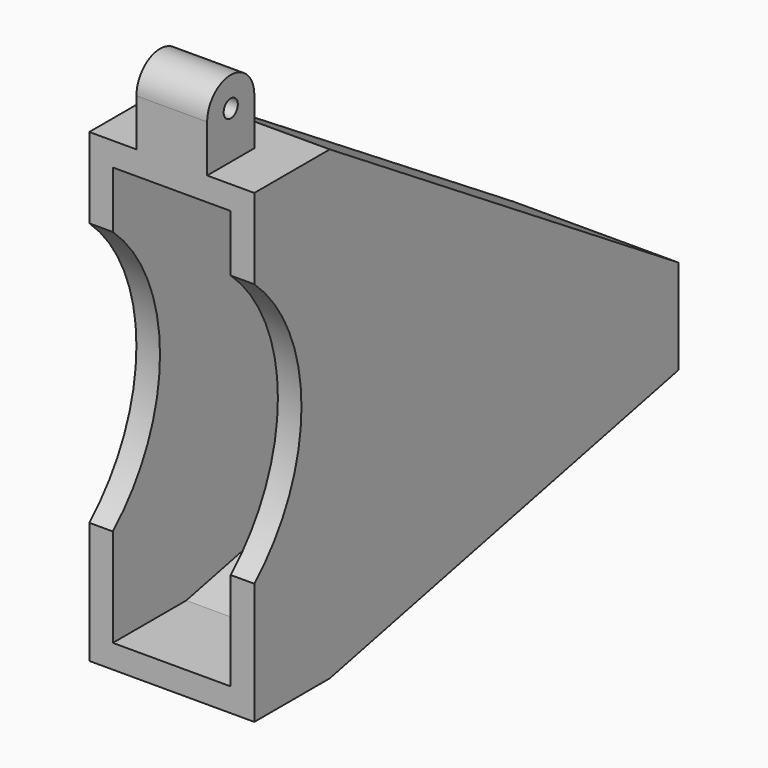
from build123d import *

# Parameters (mm, degrees)
F1_DEPTH = 7
F2_T     = -2
F3_R     = 0.75
F4_DEPTH = 3


# Not quite as in the source:
# - a feature names something its author has since deleted; it is built from what else it names


with BuildPart() as f1:
    # F0 (on Right) → F1 (new body, symmetric)
    with BuildSketch(Plane.YZ):
        with BuildLine():
            Line((45, 8), (45, 16))
            Line((45, 16), (8, 39.5))
            Line((8, 39.5), (0, 39.5))
            Line((0, 39.5), (0, 32.6803398875))
            ThreePointArc((0, 32.6803398875), (5, 21.5), (0, 10.3196601125))
            Line((0, 10.3196601125), (0, 0))
            Line((0, 0), (8, 0))
            Line((8, 0), (45, 8))
        make_face()
    extrude(amount=F1_DEPTH, both=True)

    # F2
    f2_openings = [f1.faces().sort_by_distance(p)[0] for p in [
        (0, 0, 36.09017),
        (0, 5, 21.5),
        (0, 0, 5.15983),
        (0, 45, 12),
    ]]
    offset(amount=F2_T, openings=f2_openings)

    # F3 (on Right) → F4 (join, symmetric)
    with BuildSketch(Plane.YZ):
        with BuildLine():
            Line((0, 39.5), (5, 39.5))
            Line((5, 39.5), (5, 43.5))
            ThreePointArc((5, 43.5), (2.5, 46), (0, 43.5))
            Line((0, 43.5), (0, 39.5))
        make_face()
        with Locations((2.5, 43.5)):
            Circle(F3_R, mode=Mode.SUBTRACT)
    extrude(amount=F4_DEPTH, both=True)


solid = f1.part
